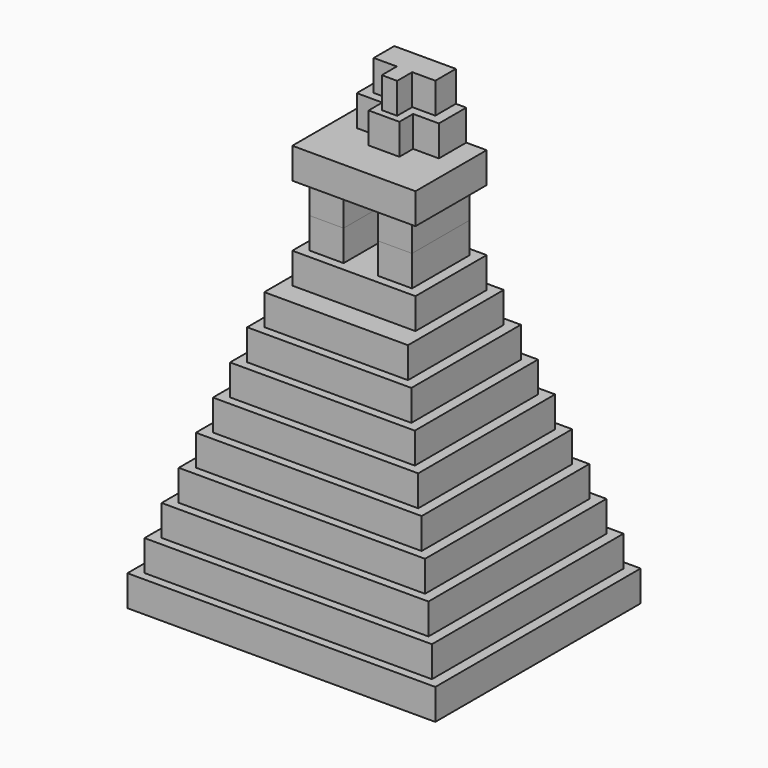
from build123d import *

# Parameters (mm, degrees)
F1_START  = -68.58
F0_W      = 76.2
F0_H      = 63.5
F0_W_2    = 71.12
F0_H_2    = 59.2666666667
F0_W_3    = 66.04
F0_H_3    = 55.0333333333
F0_W_4    = 60.96
F0_H_4    = 50.8
F0_W_5    = 55.88
F0_H_5    = 46.5666666667
F0_W_6    = 50.8
F0_H_6    = 42.3333333333
F0_W_7    = 45.72
F0_H_7    = 38.1
F0_W_8    = 40.64
F0_H_8    = 33.8666666667
F0_W_9    = 35.56
F0_H_9    = 29.6333333333
F0_W_10   = 30.48
F0_H_10   = 22.0133333333
F0_W_11   = 8.4666666667
F0_H_11   = 14.3933333333
F1_DEPTH  = 7.62
F2_START  = -60.96
F2_DEPTH  = 7.62
F3_START  = -53.34
F3_DEPTH  = 7.62
F4_START  = -45.72
F4_DEPTH  = 7.62
F5_START  = -38.1
F5_DEPTH  = 7.62
F6_START  = -30.48
F6_DEPTH  = 7.62
F7_START  = -22.86
F7_DEPTH  = 7.62
F8_START  = -15.24
F8_DEPTH  = 7.62
F9_START  = -7.62
F9_DEPTH  = 7.62
F10_DEPTH = 7.62
F11_DEPTH = 7.62
F12_START = 15.24
F12_DEPTH = 7.62
F13_W     = 1.905
F13_H     = 2.1166666667
F13_W_2   = 3.81
F13_H_2   = 6.35
F13_H_3   = 2.54
F14_DEPTH = 7.62
F15_START = 7.62
F15_DEPTH = 7.62
F16_START = 7.62
F16_DEPTH = 7.62


# Not quite as in the source:
# - a feature names something its author has since deleted; it is built from what else it names


with BuildPart() as f1:
    # F0 (on Top) → F1 (new body)
    with BuildSketch(Plane.XY.offset(F1_START)):
        Rectangle(F0_W, F0_H)
        Rectangle(F0_W_2, F0_H_2, mode=Mode.SUBTRACT)
        Rectangle(F0_W_2, F0_H_2)
        Rectangle(F0_W_3, F0_H_3, mode=Mode.SUBTRACT)
        Rectangle(F0_W_3, F0_H_3)
        Rectangle(F0_W_4, F0_H_4, mode=Mode.SUBTRACT)
        Rectangle(F0_W_4, F0_H_4)
        Rectangle(F0_W_5, F0_H_5, mode=Mode.SUBTRACT)
        Rectangle(F0_W_5, F0_H_5)
        Rectangle(F0_W_6, F0_H_6, mode=Mode.SUBTRACT)
        Rectangle(F0_W_6, F0_H_6)
        Rectangle(F0_W_7, F0_H_7, mode=Mode.SUBTRACT)
        Rectangle(F0_W_7, F0_H_7)
        Rectangle(F0_W_8, F0_H_8, mode=Mode.SUBTRACT)
        Rectangle(F0_W_8, F0_H_8)
        Rectangle(F0_W_9, F0_H_9, mode=Mode.SUBTRACT)
        Rectangle(F0_W_9, F0_H_9)
        with Locations((0, 1.6933333333)):
            Rectangle(F0_W_10, F0_H_10, mode=Mode.SUBTRACT)
        with Locations((0, 1.6933333333)):
            Rectangle(F0_W_10, F0_H_10)
        Polygon((-12.7, -7.1966666667), (-12.7, 10.5833333333), (12.7, 10.5833333333), (12.7, -7.1966666667), (4.2333333333, -7.1966666667), (-4.2333333333, -7.1966666667), align=None, mode=Mode.SUBTRACT)
        Polygon((12.7, 10.5833333333), (-12.7, 10.5833333333), (-12.7, -7.1966666667), (-4.2333333333, -7.1966666667), (-4.2333333333, 7.1966666667), (4.2333333333, 7.1966666667), (4.2333333333, -7.1966666667), (12.7, -7.1966666667), align=None)
        Rectangle(F0_W_11, F0_H_11)
    extrude(amount=-F1_DEPTH)


with BuildPart() as f2:
    # F0 (on Top) → F2 (new body)
    with BuildSketch(Plane.XY.offset(F2_START)):
        Rectangle(F0_W_2, F0_H_2)
        Rectangle(F0_W_3, F0_H_3, mode=Mode.SUBTRACT)
        Rectangle(F0_W_3, F0_H_3)
        Rectangle(F0_W_4, F0_H_4, mode=Mode.SUBTRACT)
        Rectangle(F0_W_4, F0_H_4)
        Rectangle(F0_W_5, F0_H_5, mode=Mode.SUBTRACT)
        Rectangle(F0_W_5, F0_H_5)
        Rectangle(F0_W_6, F0_H_6, mode=Mode.SUBTRACT)
        Rectangle(F0_W_6, F0_H_6)
        Rectangle(F0_W_7, F0_H_7, mode=Mode.SUBTRACT)
        Rectangle(F0_W_7, F0_H_7)
        Rectangle(F0_W_8, F0_H_8, mode=Mode.SUBTRACT)
        Rectangle(F0_W_8, F0_H_8)
        Rectangle(F0_W_9, F0_H_9, mode=Mode.SUBTRACT)
        Rectangle(F0_W_9, F0_H_9)
        with Locations((0, 1.6933333333)):
            Rectangle(F0_W_10, F0_H_10, mode=Mode.SUBTRACT)
        with Locations((0, 1.6933333333)):
            Rectangle(F0_W_10, F0_H_10)
        Polygon((-12.7, -7.1966666667), (-12.7, 10.5833333333), (12.7, 10.5833333333), (12.7, -7.1966666667), (4.2333333333, -7.1966666667), (-4.2333333333, -7.1966666667), align=None, mode=Mode.SUBTRACT)
        Polygon((12.7, 10.5833333333), (-12.7, 10.5833333333), (-12.7, -7.1966666667), (-4.2333333333, -7.1966666667), (-4.2333333333, 7.1966666667), (4.2333333333, 7.1966666667), (4.2333333333, -7.1966666667), (12.7, -7.1966666667), align=None)
        Rectangle(F0_W_11, F0_H_11)
    extrude(amount=-F2_DEPTH)


with BuildPart() as f3:
    # F0 (on Top) → F3 (new body)
    with BuildSketch(Plane.XY.offset(F3_START)):
        Rectangle(F0_W_3, F0_H_3)
        Rectangle(F0_W_4, F0_H_4, mode=Mode.SUBTRACT)
        Rectangle(F0_W_4, F0_H_4)
        Rectangle(F0_W_5, F0_H_5, mode=Mode.SUBTRACT)
        Rectangle(F0_W_5, F0_H_5)
        Rectangle(F0_W_6, F0_H_6, mode=Mode.SUBTRACT)
        Rectangle(F0_W_6, F0_H_6)
        Rectangle(F0_W_7, F0_H_7, mode=Mode.SUBTRACT)
        Rectangle(F0_W_7, F0_H_7)
        Rectangle(F0_W_8, F0_H_8, mode=Mode.SUBTRACT)
        Rectangle(F0_W_8, F0_H_8)
        Rectangle(F0_W_9, F0_H_9, mode=Mode.SUBTRACT)
        Rectangle(F0_W_9, F0_H_9)
        with Locations((0, 1.6933333333)):
            Rectangle(F0_W_10, F0_H_10, mode=Mode.SUBTRACT)
        with Locations((0, 1.6933333333)):
            Rectangle(F0_W_10, F0_H_10)
        Polygon((-12.7, -7.1966666667), (-12.7, 10.5833333333), (12.7, 10.5833333333), (12.7, -7.1966666667), (4.2333333333, -7.1966666667), (-4.2333333333, -7.1966666667), align=None, mode=Mode.SUBTRACT)
        Polygon((12.7, 10.5833333333), (-12.7, 10.5833333333), (-12.7, -7.1966666667), (-4.2333333333, -7.1966666667), (-4.2333333333, 7.1966666667), (4.2333333333, 7.1966666667), (4.2333333333, -7.1966666667), (12.7, -7.1966666667), align=None)
        Rectangle(F0_W_11, F0_H_11)
    extrude(amount=-F3_DEPTH)


with BuildPart() as f4:
    # F0 (on Top) → F4 (new body)
    with BuildSketch(Plane.XY.offset(F4_START)):
        Rectangle(F0_W_4, F0_H_4)
        Rectangle(F0_W_5, F0_H_5, mode=Mode.SUBTRACT)
        Rectangle(F0_W_5, F0_H_5)
        Rectangle(F0_W_6, F0_H_6, mode=Mode.SUBTRACT)
        Rectangle(F0_W_6, F0_H_6)
        Rectangle(F0_W_7, F0_H_7, mode=Mode.SUBTRACT)
        Rectangle(F0_W_7, F0_H_7)
        Rectangle(F0_W_8, F0_H_8, mode=Mode.SUBTRACT)
        Rectangle(F0_W_8, F0_H_8)
        Rectangle(F0_W_9, F0_H_9, mode=Mode.SUBTRACT)
        Rectangle(F0_W_9, F0_H_9)
        with Locations((0, 1.6933333333)):
            Rectangle(F0_W_10, F0_H_10, mode=Mode.SUBTRACT)
        with Locations((0, 1.6933333333)):
            Rectangle(F0_W_10, F0_H_10)
        Polygon((-12.7, -7.1966666667), (-12.7, 10.5833333333), (12.7, 10.5833333333), (12.7, -7.1966666667), (4.2333333333, -7.1966666667), (-4.2333333333, -7.1966666667), align=None, mode=Mode.SUBTRACT)
        Polygon((12.7, 10.5833333333), (-12.7, 10.5833333333), (-12.7, -7.1966666667), (-4.2333333333, -7.1966666667), (-4.2333333333, 7.1966666667), (4.2333333333, 7.1966666667), (4.2333333333, -7.1966666667), (12.7, -7.1966666667), align=None)
        Rectangle(F0_W_11, F0_H_11)
    extrude(amount=-F4_DEPTH)


with BuildPart() as f5:
    # F0 (on Top) → F5 (new body)
    with BuildSketch(Plane.XY.offset(F5_START)):
        Rectangle(F0_W_5, F0_H_5)
        Rectangle(F0_W_6, F0_H_6, mode=Mode.SUBTRACT)
        Rectangle(F0_W_6, F0_H_6)
        Rectangle(F0_W_7, F0_H_7, mode=Mode.SUBTRACT)
        Rectangle(F0_W_7, F0_H_7)
        Rectangle(F0_W_8, F0_H_8, mode=Mode.SUBTRACT)
        Rectangle(F0_W_8, F0_H_8)
        Rectangle(F0_W_9, F0_H_9, mode=Mode.SUBTRACT)
        Rectangle(F0_W_9, F0_H_9)
        with Locations((0, 1.6933333333)):
            Rectangle(F0_W_10, F0_H_10, mode=Mode.SUBTRACT)
        with Locations((0, 1.6933333333)):
            Rectangle(F0_W_10, F0_H_10)
        Polygon((-12.7, -7.1966666667), (-12.7, 10.5833333333), (12.7, 10.5833333333), (12.7, -7.1966666667), (4.2333333333, -7.1966666667), (-4.2333333333, -7.1966666667), align=None, mode=Mode.SUBTRACT)
        Rectangle(F0_W_11, F0_H_11)
        Polygon((12.7, 10.5833333333), (-12.7, 10.5833333333), (-12.7, -7.1966666667), (-4.2333333333, -7.1966666667), (-4.2333333333, 7.1966666667), (4.2333333333, 7.1966666667), (4.2333333333, -7.1966666667), (12.7, -7.1966666667), align=None)
    extrude(amount=-F5_DEPTH)


with BuildPart() as f6:
    # F0 (on Top) → F6 (new body)
    with BuildSketch(Plane.XY.offset(F6_START)):
        Rectangle(F0_W_6, F0_H_6)
        Rectangle(F0_W_7, F0_H_7, mode=Mode.SUBTRACT)
        Rectangle(F0_W_7, F0_H_7)
        Rectangle(F0_W_8, F0_H_8, mode=Mode.SUBTRACT)
        Rectangle(F0_W_8, F0_H_8)
        Rectangle(F0_W_9, F0_H_9, mode=Mode.SUBTRACT)
        Rectangle(F0_W_9, F0_H_9)
        with Locations((0, 1.6933333333)):
            Rectangle(F0_W_10, F0_H_10, mode=Mode.SUBTRACT)
        with Locations((0, 1.6933333333)):
            Rectangle(F0_W_10, F0_H_10)
        Polygon((-12.7, -7.1966666667), (-12.7, 10.5833333333), (12.7, 10.5833333333), (12.7, -7.1966666667), (4.2333333333, -7.1966666667), (-4.2333333333, -7.1966666667), align=None, mode=Mode.SUBTRACT)
        Polygon((12.7, 10.5833333333), (-12.7, 10.5833333333), (-12.7, -7.1966666667), (-4.2333333333, -7.1966666667), (-4.2333333333, 7.1966666667), (4.2333333333, 7.1966666667), (4.2333333333, -7.1966666667), (12.7, -7.1966666667), align=None)
        Rectangle(F0_W_11, F0_H_11)
    extrude(amount=-F6_DEPTH)


with BuildPart() as f7:
    # F0 (on Top) → F7 (new body)
    with BuildSketch(Plane.XY.offset(F7_START)):
        Rectangle(F0_W_7, F0_H_7)
        Rectangle(F0_W_8, F0_H_8, mode=Mode.SUBTRACT)
        Rectangle(F0_W_8, F0_H_8)
        Rectangle(F0_W_9, F0_H_9, mode=Mode.SUBTRACT)
        Rectangle(F0_W_9, F0_H_9)
        with Locations((0, 1.6933333333)):
            Rectangle(F0_W_10, F0_H_10, mode=Mode.SUBTRACT)
        with Locations((0, 1.6933333333)):
            Rectangle(F0_W_10, F0_H_10)
        Polygon((-12.7, -7.1966666667), (-12.7, 10.5833333333), (12.7, 10.5833333333), (12.7, -7.1966666667), (4.2333333333, -7.1966666667), (-4.2333333333, -7.1966666667), align=None, mode=Mode.SUBTRACT)
        Polygon((12.7, 10.5833333333), (-12.7, 10.5833333333), (-12.7, -7.1966666667), (-4.2333333333, -7.1966666667), (-4.2333333333, 7.1966666667), (4.2333333333, 7.1966666667), (4.2333333333, -7.1966666667), (12.7, -7.1966666667), align=None)
        Rectangle(F0_W_11, F0_H_11)
    extrude(amount=-F7_DEPTH)


with BuildPart() as f8:
    # F0 (on Top) → F8 (new body)
    with BuildSketch(Plane.XY.offset(F8_START)):
        Rectangle(F0_W_8, F0_H_8)
        Rectangle(F0_W_9, F0_H_9, mode=Mode.SUBTRACT)
        Rectangle(F0_W_9, F0_H_9)
        with Locations((0, 1.6933333333)):
            Rectangle(F0_W_10, F0_H_10, mode=Mode.SUBTRACT)
        with Locations((0, 1.6933333333)):
            Rectangle(F0_W_10, F0_H_10)
        Polygon((-12.7, -7.1966666667), (-12.7, 10.5833333333), (12.7, 10.5833333333), (12.7, -7.1966666667), (4.2333333333, -7.1966666667), (-4.2333333333, -7.1966666667), align=None, mode=Mode.SUBTRACT)
        Polygon((12.7, 10.5833333333), (-12.7, 10.5833333333), (-12.7, -7.1966666667), (-4.2333333333, -7.1966666667), (-4.2333333333, 7.1966666667), (4.2333333333, 7.1966666667), (4.2333333333, -7.1966666667), (12.7, -7.1966666667), align=None)
        Rectangle(F0_W_11, F0_H_11)
    extrude(amount=-F8_DEPTH)


with BuildPart() as f9:
    # F0 (on Top) → F9 (new body)
    with BuildSketch(Plane.XY.offset(F9_START)):
        Rectangle(F0_W_9, F0_H_9)
        with Locations((0, 1.6933333333)):
            Rectangle(F0_W_10, F0_H_10, mode=Mode.SUBTRACT)
        with Locations((0, 1.6933333333)):
            Rectangle(F0_W_10, F0_H_10)
        Polygon((-12.7, -7.1966666667), (-12.7, 10.5833333333), (12.7, 10.5833333333), (12.7, -7.1966666667), (4.2333333333, -7.1966666667), (-4.2333333333, -7.1966666667), align=None, mode=Mode.SUBTRACT)
        Polygon((12.7, 10.5833333333), (-12.7, 10.5833333333), (-12.7, -7.1966666667), (-4.2333333333, -7.1966666667), (-4.2333333333, 7.1966666667), (4.2333333333, 7.1966666667), (4.2333333333, -7.1966666667), (12.7, -7.1966666667), align=None)
        Rectangle(F0_W_11, F0_H_11)
    extrude(amount=-F9_DEPTH)


with BuildPart() as f10:
    # F0 (on Top) → F10 (new body)
    with BuildSketch(Plane.XY):
        with Locations((0, 1.6933333333)):
            Rectangle(F0_W_10, F0_H_10)
        Polygon((-12.7, -7.1966666667), (-12.7, 10.5833333333), (12.7, 10.5833333333), (12.7, -7.1966666667), (4.2333333333, -7.1966666667), (-4.2333333333, -7.1966666667), align=None, mode=Mode.SUBTRACT)
        Polygon((12.7, 10.5833333333), (-12.7, 10.5833333333), (-12.7, -7.1966666667), (-4.2333333333, -7.1966666667), (-4.2333333333, 7.1966666667), (4.2333333333, 7.1966666667), (4.2333333333, -7.1966666667), (12.7, -7.1966666667), align=None)
        Rectangle(F0_W_11, F0_H_11)
    extrude(amount=-F10_DEPTH)


with BuildPart() as f11:
    # F0 (on Top) → F11 (new body)
    with BuildSketch(Plane.XY):
        Polygon((12.7, 10.5833333333), (-12.7, 10.5833333333), (-12.7, -7.1966666667), (-4.2333333333, -7.1966666667), (-4.2333333333, 7.1966666667), (4.2333333333, 7.1966666667), (4.2333333333, -7.1966666667), (12.7, -7.1966666667), align=None)
    extrude(amount=F11_DEPTH)


with BuildPart() as f12:
    # F0 (on Top) → F12 (new body)
    with BuildSketch(Plane.XY.offset(F12_START)):
        with Locations((0, 1.6933333333)):
            Rectangle(F0_W_10, F0_H_10)
        Polygon((-12.7, -7.1966666667), (-12.7, 10.5833333333), (12.7, 10.5833333333), (12.7, -7.1966666667), (4.2333333333, -7.1966666667), (-4.2333333333, -7.1966666667), align=None, mode=Mode.SUBTRACT)
        Polygon((12.7, 10.5833333333), (-12.7, 10.5833333333), (-12.7, -7.1966666667), (-4.2333333333, -7.1966666667), (-4.2333333333, 7.1966666667), (4.2333333333, 7.1966666667), (4.2333333333, -7.1966666667), (12.7, -7.1966666667), align=None)
        Rectangle(F0_W_11, F0_H_11)
    extrude(amount=F12_DEPTH)


with BuildPart() as f14:
    # F13 (on face) → F14 (new body)
    with BuildSketch(Plane.XY.offset(22.86)):
        Polygon((-7.62, 12.7), (-10.1297069341, 12.7), (-10.1297069341, 4.2333333333), (-3.81, 4.2333333333), (-3.81, 6.35), (-7.62, 6.35), align=None)
        with Locations((2.8575, 5.2916666667)):
            Rectangle(F13_W, F13_H)
        with Locations((-2.8575, 5.2916666667)):
            Rectangle(F13_W, F13_H)
        Polygon((-1.905, 4.2333333333), (-3.81, 4.2333333333), (-3.81, 0), (3.81, 0), (3.81, 4.2333333333), (1.905, 4.2333333333), (1.905, 1.6933333333), (-1.905, 1.6933333333), align=None)
        Polygon((3.81, 6.35), (3.81, 4.2333333333), (10.1902930659, 4.2333333333), (10.1902930659, 12.7), (7.62, 12.7), (7.62, 6.35), align=None)
        with Locations((5.715, 9.525)):
            Rectangle(F13_W_2, F13_H_2)
        with Locations((2.8575, 9.525)):
            Rectangle(F13_W, F13_H_2)
        with Locations((0, 9.525)):
            Rectangle(F13_W_2, F13_H_2)
        with Locations((0, 5.2916666667)):
            Rectangle(F13_W_2, F13_H)
        with Locations((0, 2.9633333333)):
            Rectangle(F13_W_2, F13_H_3)
        with Locations((-2.8575, 9.525)):
            Rectangle(F13_W, F13_H_2)
        with Locations((-5.715, 9.525)):
            Rectangle(F13_W_2, F13_H_2)
    extrude(amount=F14_DEPTH)


with BuildPart() as f15:
    # F13 (on face) → F15 (new body)
    with BuildSketch(Plane.XY.offset(22.86).offset(F15_START)):
        with Locations((-5.715, 9.525)):
            Rectangle(F13_W_2, F13_H_2)
        with Locations((-2.8575, 9.525)):
            Rectangle(F13_W, F13_H_2)
        with Locations((0, 9.525)):
            Rectangle(F13_W_2, F13_H_2)
        with Locations((2.8575, 9.525)):
            Rectangle(F13_W, F13_H_2)
        with Locations((5.715, 9.525)):
            Rectangle(F13_W_2, F13_H_2)
        with Locations((0, 5.2916666667)):
            Rectangle(F13_W_2, F13_H)
        with Locations((0, 2.9633333333)):
            Rectangle(F13_W_2, F13_H_3)
    extrude(amount=F15_DEPTH)


with BuildPart() as f16:
    # F0 (on Top) → F16 (new body)
    with BuildSketch(Plane.XY.offset(F16_START)):
        Polygon((12.7, 10.5833333333), (-12.7, 10.5833333333), (-12.7, -7.1966666667), (-4.2333333333, -7.1966666667), (-4.2333333333, 7.1966666667), (4.2333333333, 7.1966666667), (4.2333333333, -7.1966666667), (12.7, -7.1966666667), align=None)
    extrude(amount=F16_DEPTH)


solid = Compound([f1.part, f2.part, f3.part, f4.part, f5.part, f6.part, f7.part, f8.part, f9.part, f10.part, f11.part, f12.part, f14.part, f15.part, f16.part])
